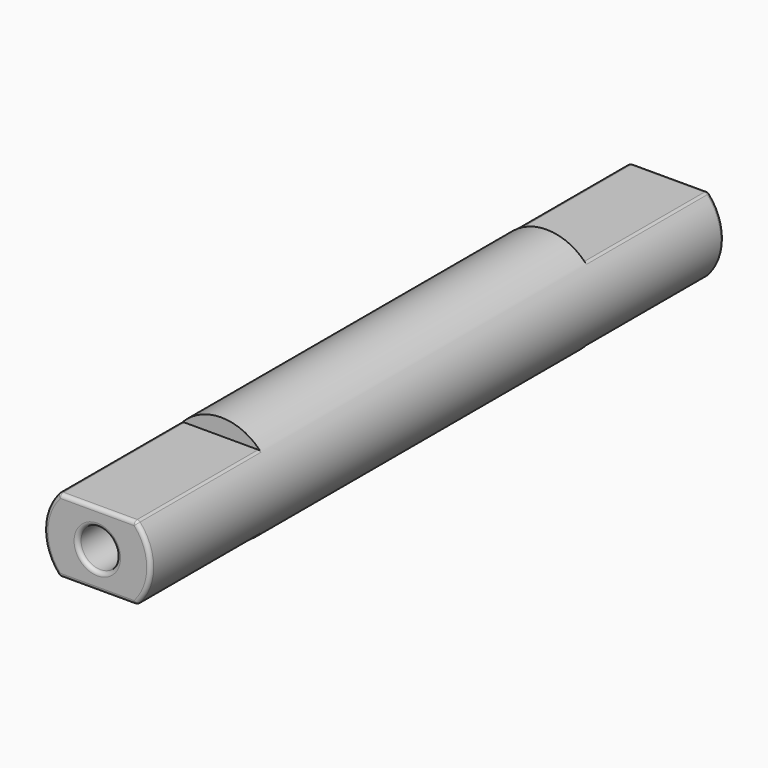
from build123d import *

# Parameters (mm, degrees)
F0_R           = 2.75
F1_DEPTH       = 18.5
F3_DEPTH       = 8
F7_D           = 2
F7_DEPTH       = 6
F7_TIP         = 0.600860619
F7_ON_F5_D     = 2
F7_ON_F5_DEPTH = 6
F7_ON_F5_TIP   = 0.600860619
F8_R           = 0.2


with BuildPart() as f1:
    # F0 (on Front) → F1 (new body, symmetric)
    with BuildSketch(Plane.XZ):
        Circle(F0_R)
    extrude(amount=F1_DEPTH, both=True)

    # F2 (on face) → F3 (cut)
    with BuildSketch(Plane.XZ.offset(18.5)):
        with BuildLine():
            ThreePointArc((1.9880895352, 1.9), (1.0810874155, 2.5285865617), (0, 2.75))
            ThreePointArc((0, 2.75), (-1.0810874155, 2.5285865617), (-1.9880895352, 1.9))
            Line((-1.9880895352, 1.9), (1.9880895352, 1.9))
        make_face()
        with BuildLine():
            Line((1.9880895352, -1.9), (-1.9880895352, -1.9))
            ThreePointArc((-1.9880895352, -1.9), (-1.0810874155, -2.5285865617), (0, -2.75))
            ThreePointArc((0, -2.75), (1.0810874155, -2.5285865617), (1.9880895352, -1.9))
        make_face()
    extrude(amount=-F3_DEPTH, mode=Mode.SUBTRACT)

    # F4: F1 across plane


with BuildPart() as f1_1:
    add(f1.part)
    add(f1.part.mirror(Plane.XZ), mode=Mode.INTERSECT)

    # F7
    with Locations(Plane(origin=(0, 18.5, 0), x_dir=(-1, 0, 0), z_dir=(0, 1, 0))):
        with Locations((0, 0)):
            Hole(F7_D / 2, depth=F7_DEPTH)
            with Locations((0, 0, -(F7_DEPTH + F7_TIP / 2))):  # 118° drill point
                Cone(0, F7_D / 2, F7_TIP, mode=Mode.SUBTRACT)

    # F7 on F5
    with Locations(Plane.XZ.offset(18.5)):
        with Locations((0, 0)):
            Hole(F7_ON_F5_D / 2, depth=F7_ON_F5_DEPTH)
            with Locations((0, 0, -(F7_ON_F5_DEPTH + F7_ON_F5_TIP / 2))):  # 118° drill point
                Cone(0, F7_ON_F5_D / 2, F7_ON_F5_TIP, mode=Mode.SUBTRACT)

    # F8
    f8_edges = [f1_1.edges().sort_by_distance(p)[0] for p in [
        (2.552425, -18.5, 1.023536),
        (-2.75, -18.5, 0),
        (2.552425, -18.5, -1.023536),
        (-1.98809, -14.5, -1.9),
        (1.98809, -14.5, -1.9),
        (1.98809, -14.5, 1.9),
        (-1.98809, -14.5, 1.9),
        (0, -18.5, -1.9),
        (0, -18.5, 1.9),
        (1.98809, 14.5, 1.9),
        (-1.98809, 14.5, 1.9),
        (-1.98809, 14.5, -1.9),
        (1.98809, 14.5, -1.9),
        (2.552425, 18.5, -1.023536),
        (0, 18.5, -1.9),
        (2.552425, 18.5, 1.023536),
        (-2.75, 18.5, 0),
        (0, 18.5, 1.9),
        (1, 18.5, 0),
        (-1, -18.5, 0),
    ]]
    fillet(f8_edges, radius=F8_R)


solid = f1_1.part
